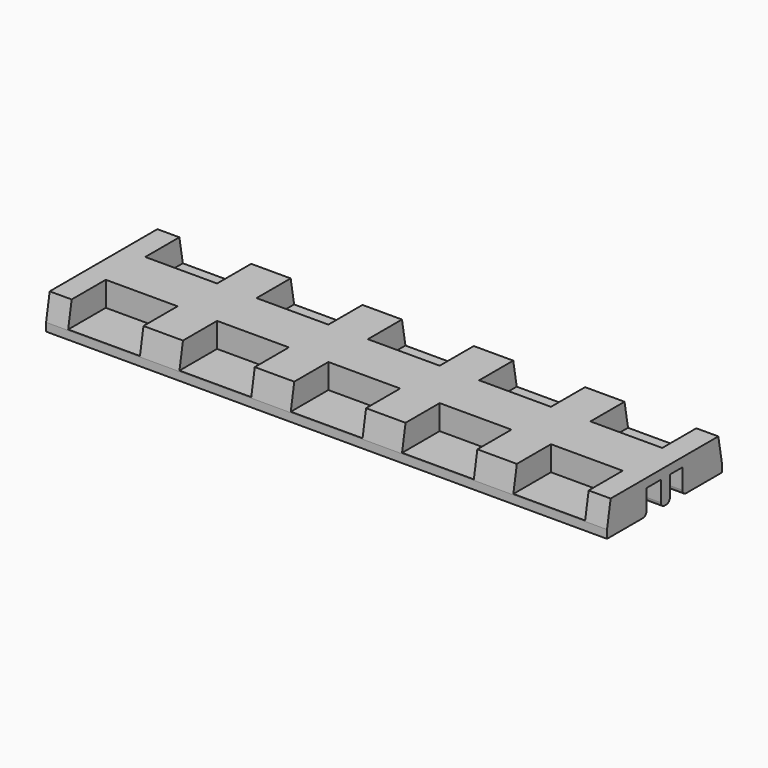
from build123d import *

# Parameters (mm, degrees)
F1_DEPTH    = 5.5
F2_W        = 125
F2_H        = 32
F3_DEPTH    = 2
F4_W        = 3.5
F4_H        = 5.5
F4_W_2      = 4
F5_DEPTH    = 125
F6_R        = 1
F7_C1_SIZE2 = 1
F7_C1_SIZE  = 5.6712818196
F7_C2_SIZE2 = 5.6712818196
F7_C2_SIZE  = 1


with BuildPart() as f1:
    # F0 (on Top) → F1 (new body)
    with BuildSketch(Plane.XY):
        Polygon((57.6, -16.5), (62.5, -16.5), (62.5, 15.5), (57.6, 15.5), (57.6, 5), (41.6, 5), (41.6, 15.5), (32.8, 15.5), (32.8, 5), (16.8, 5), (16.8, 15.5), (8, 15.5), (8, 5), (-8, 5), (-8, 15.5), (-16.8, 15.5), (-16.8, 5), (-32.8, 5), (-32.8, 15.5), (-41.6, 15.5), (-41.6, 5), (-57.6, 5), (-57.6, 15.5), (-62.5, 15.5), (-62.5, -16.5), (-57.6, -16.5), (-57.6, -6), (-41.6, -6), (-41.6, -16.5), (-32.8, -16.5), (-32.8, -6), (-16.8, -6), (-16.8, -16.5), (-8, -16.5), (-8, -6), (8, -6), (8, -16.5), (16.8, -16.5), (16.8, -6), (32.8, -6), (32.8, -16.5), (41.6, -16.5), (41.6, -6), (57.6, -6), align=None)
    extrude(amount=F1_DEPTH)

    # F2 (on face) → F3 (join)
    with BuildSketch(Plane(origin=(0, 0, 0), x_dir=(1, 0, 0), z_dir=(0, 0, -1))):
        with Locations((0, 0.5)):
            Rectangle(F2_W, F2_H)
    extrude(amount=F3_DEPTH)

    # F4 (on face) → F5 (cut, through all)
    with BuildSketch(Plane(origin=(-62.5, 0, 0), x_dir=(0, -1, 0), z_dir=(-1, 0, 0))):
        with Locations((-2.75, 0.75)):
            Rectangle(F4_W, F4_H)
        with Locations((3.5, 0.75)):
            Rectangle(F4_W_2, F4_H)
    extrude(amount=-F5_DEPTH, mode=Mode.SUBTRACT)

    # F6
    f6_edges = [f1.edges().sort_by_distance(p)[0] for p in [
        (0, 4.5, -2),
        (0, 1, -2),
        (0, -5.5, -2),
        (0, -1.5, -2),
    ]]
    fillet(f6_edges, radius=F6_R)

    # F7: chamfer of 1 x 5.6712818196 on 12 edges, made by hand

    # F7_c1
    f7_c1_edges = [f1.edges().sort_by_distance(p)[0] for p in [
        (-12.4, -16.5, 5.5),
    ]]
    f7_c1_side = f1.faces().sort_by_distance((-12.4, -16.5, 5.48))[0]
    chamfer(f7_c1_edges, length=F7_C1_SIZE, length2=F7_C1_SIZE2, reference=f7_c1_side)

    # F7_c2
    f7_c2_edges = [f1.edges().sort_by_distance(p)[0] for p in [
        (12.4, 15.5, 5.5),
    ]]
    f7_c2_side = f1.faces().sort_by_distance((12.4, 15.48, 5.5))[0]
    chamfer(f7_c2_edges, length=F7_C2_SIZE, length2=F7_C2_SIZE2, reference=f7_c2_side)


solid = f1.part
